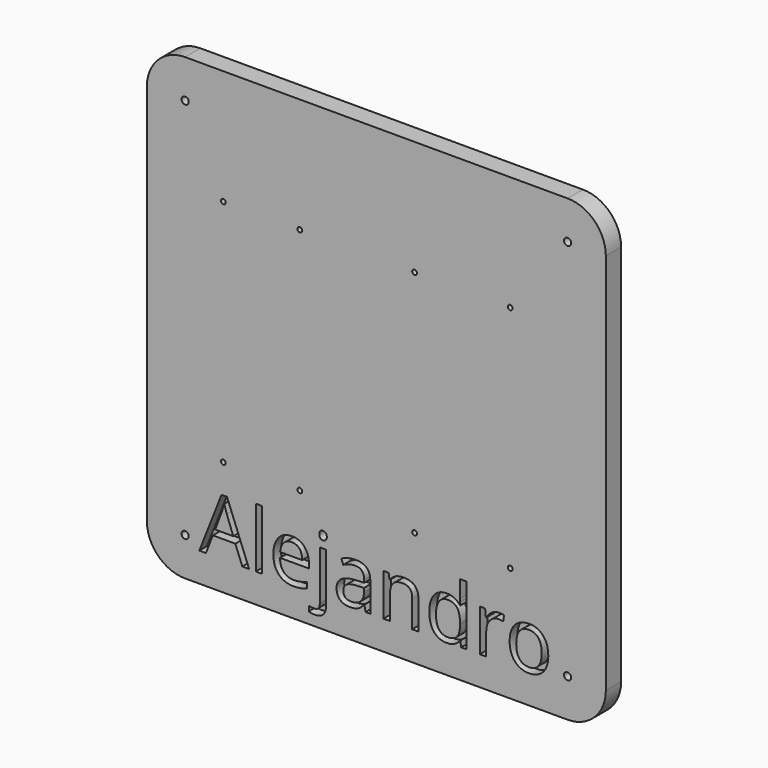
from build123d import *

# Parameters (mm, degrees)
F0_W         = 304.8
F0_H         = 304.8
F1_DEPTH     = 12.7
F3_D         = 3.175
F5_D         = 4.7752
F6_R         = 25.4
F7_TEXT_SIZE = 52.2111111111
F8_DEPTH     = 6.35


# Not quite as in the source:
# - Text() gives the source's letters only with a copy of the font that has no kerning and outlines rounded to 1/6400 em; it was checked with that copy


with BuildPart() as f1:
    # F0 (on Front) → F1 (new body)
    with BuildSketch(Plane.XZ):
        with Locations((143.9738112075, 152.4)):
            Rectangle(F0_W, F0_H)
    extrude(amount=F1_DEPTH)

    # F3 (through all)
    with Locations(Plane.XZ.offset(12.7)):
        with Locations((42.3738112075, 228.6), (93.1738112075, 228.6), (169.3738112075, 228.6), (232.8738112075, 228.6), (42.3738112075, 76.2), (93.1738112075, 76.2), (169.3738112075, 76.2), (232.8738112075, 76.2)):
            Hole(F3_D / 2)

    # F5 (through all)
    with Locations(Plane.XZ.offset(12.7)):
        with Locations((16.9738112075, 279.4), (270.9738112075, 279.4), (16.9738112075, 25.4), (270.9738112075, 25.4)):
            Hole(F5_D / 2)

    # F6
    f6_edges = [f1.edges().sort_by_distance(p)[0] for p in [
        (-8.426189, -6.35, 304.8),
        (296.373811, -6.35, 304.8),
        (296.373811, -6.35, 0),
        (-8.426189, -6.35, 0),
    ]]
    fillet(f6_edges, radius=F6_R)

    # F7 (on face) → F8 (cut)
    with BuildSketch(Plane.XZ.offset(12.7)):
        with Locations((26.4090733603, 19.3330312119)):
            Text('Alejandro', F7_TEXT_SIZE, font='Open Sans', text_align=(TextAlign.LEFT, TextAlign.BOTTOM))
    extrude(amount=-F8_DEPTH, mode=Mode.SUBTRACT)


solid = f1.part
